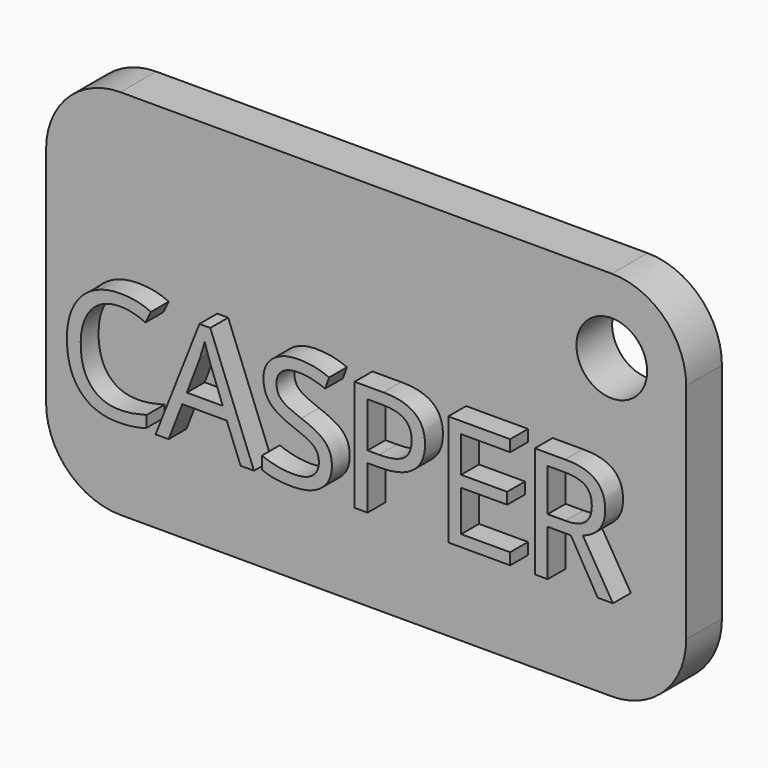
from build123d import *

# Parameters (mm, degrees)
F1_DEPTH     = 3
F2_R         = 2.3741230432
F3_DEPTH     = 3
F4_TEXT_SIZE = 10.4489795918
F5_DEPTH     = 1.5


# Not quite as in the source:
# - Text() gives the source's letters only with a copy of the font that has no kerning and outlines rounded to 1/6400 em; it was checked with that copy


with BuildPart() as f1:
    # F0 (on Front) → F1 (new body)
    with BuildSketch(Plane.XZ):
        with BuildLine():
            ThreePointArc((0, 5), (1.4644660941, 1.4644660941), (5, 0))
            Line((5, 0), (38, 0))
            ThreePointArc((38, 0), (41.5355339059, 1.4644660941), (43, 5))
            Line((43, 5), (43, 20))
            ThreePointArc((43, 20), (41.5355339059, 23.5355339059), (38, 25))
            Line((38, 25), (5, 25))
            ThreePointArc((5, 25), (1.4644660941, 23.5355339059), (0, 20))
            Line((0, 20), (0, 5))
        make_face()
    extrude(amount=F1_DEPTH)

    # F2 (on face) → F3 (cut)
    with BuildSketch(Plane.XZ.offset(3)):
        with Locations((38, 20)):
            Circle(F2_R)
    extrude(amount=-F3_DEPTH, mode=Mode.SUBTRACT)

    # F4 (on face) → F5 (join)
    with BuildSketch(Plane.XZ.offset(3)):
        with Locations((1.9602822228, 6.5305768093)):
            Text('CASPER', F4_TEXT_SIZE, font='Open Sans', text_align=(TextAlign.LEFT, TextAlign.BOTTOM))
    extrude(amount=F5_DEPTH)


solid = f1.part
